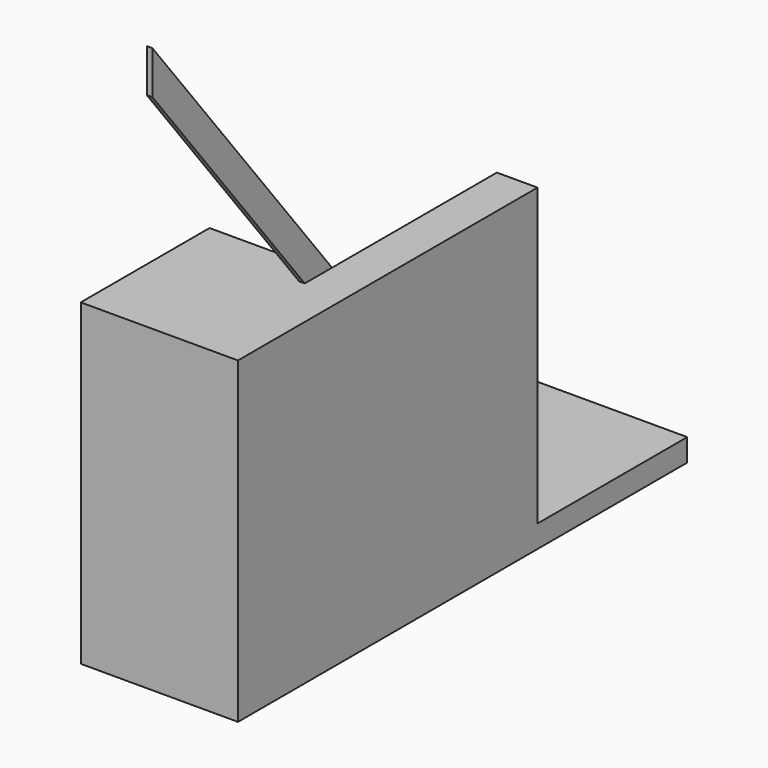
from build123d import *

# Parameters (mm, degrees)
F0_W      = 2000
F0_H      = 2000
F1_DEPTH  = 1500
F2_W      = 1782.87
F2_H      = 1480
F3_DEPTH  = 1140
F5_DEPTH  = 1000
F6_DEPTH  = 200
F8_DEPTH  = 100
F10_DEPTH = 200
F11_DEPTH = 200
F12_DEPTH = 63.2839202881
F13_W     = 115
F13_H     = 85
F14_DEPTH = 30
F16_DEPTH = 1360
F18_DEPTH = 30


with BuildPart() as f1:
    # F0 (on Top) → F1 (new body)
    with BuildSketch(Plane.XY):
        with Locations((1000, 1000)):
            Rectangle(F0_W, F0_H)
    extrude(amount=F1_DEPTH)

    # F2 (on face) → F3 (cut)
    with BuildSketch(Plane(origin=(0, 2000, 0), x_dir=(-1, 0, 0), z_dir=(0, 1, 0))):
        with Locations((-891.435, 760)):
            Rectangle(F2_W, F2_H)
    extrude(amount=-F3_DEPTH, mode=Mode.SUBTRACT)

    # F4 (on face) → F5 (join)
    with BuildSketch(Plane(origin=(0, 2000, 0), x_dir=(-1, 0, 0), z_dir=(0, 1, 0))):
        Polygon((-2000, 0), (0, 0), (0, 20), (-1782.87, 20), (-2000, 20), align=None)
    extrude(amount=F5_DEPTH)

    # F6 (add): a face of the model
    f6_faces = [f1.faces().sort_by_distance(p)[0] for p in [
        (1000, 1500, 0),
    ]]
    extrude(f6_faces, amount=F6_DEPTH)

    # F7 (on face) → F8 (cut)
    with BuildSketch(Plane.XY.offset(20)):
        Polygon((2000, 2000), (2000, 3000), (0, 3000), (0, 2000), (1782.87, 2000), align=None)
    extrude(amount=-F8_DEPTH, mode=Mode.SUBTRACT)

    # F9 (on face) → F10 (join)
    with BuildSketch(Plane(origin=(0, 0, 0), x_dir=(0, -1, 0), z_dir=(-1, 0, 0))):
        Polygon((-860, 1500), (0, 1500), (0, 1563.2839202881), (-2000, 1563.2839202881), (-2000, 20), (-860, 20), align=None)
        Polygon((-2000, -200), (0, -200), (0, 1500), (-860, 1500), (-860, 20), (-2000, 20), (-2000, -80), align=None)
    extrude(amount=F10_DEPTH)

    # F11 (add, through all): a face of the model
    f11_faces = [f1.faces().sort_by_distance(p)[0] for p in [
        (0, 2500, -140),
    ]]
    extrude(f11_faces, amount=F11_DEPTH)

    # F12 (cut, through all): a face of the model
    f12_faces = [f1.faces().sort_by_distance(p)[0] for p in [
        (-100, 1000, 1563.2839202881),
    ]]
    extrude(f12_faces, amount=-F12_DEPTH, mode=Mode.SUBTRACT)

    # F16 (cut): a face of the model
    f16_faces = [f1.faces().sort_by_distance(p)[0] for p in [
        (-200, 1051.1363636364, 623.0681818182),
    ]]
    extrude(f16_faces, amount=-F16_DEPTH, mode=Mode.SUBTRACT)


with BuildPart() as f14:
    # F13 (on face) → F14 (new body)
    with BuildSketch(Plane(origin=(-200, 0, 0), x_dir=(0, -1, 0), z_dir=(-1, 0, 0))):
        Polygon((-843.6620926244, 1500), (0, 2569.25), (0, 2654.25), (0, 2800), (-1025.7289879931, 1500), align=None)
        Polygon((-2000, 34.4673913043), (-843.6620926244, 1500), (-1025.7289879931, 1500), (-2000, 265.2173913043), align=None)
        Polygon((-2272.384219554, -80), (-2090.3173241852, -80), (-2000, 34.4673913043), (-2000, 265.2173913043), align=None)
        Polygon((-2185, -115), (-2185, -200), (-2090.3173241852, -80), (-2272.384219554, -80), (-2300, -115), align=None)
        with Locations((-2242.5, -157.5)):
            Rectangle(F13_W, F13_H)
    extrude(amount=F14_DEPTH)


with BuildPart() as f14_1:
    # F15: moved
    add(f14.part.moved(Location((1982.87, -300, 220))))


with BuildPart() as f18:
    # F17 (on face) → F18 (new body)
    with BuildSketch(Plane(origin=(1752.87, 0, 0), x_dir=(0, -1, 0), z_dir=(-1, 0, 0))):
        Polygon((-1885, 20), (-860, 1319.0760869565), (-860, 1500), (-899.3138936535, 1500), (-2000, 105), (-2000, 20), align=None)
    extrude(amount=F18_DEPTH)


solid = Compound([f1.part, f14_1.part, f18.part])
